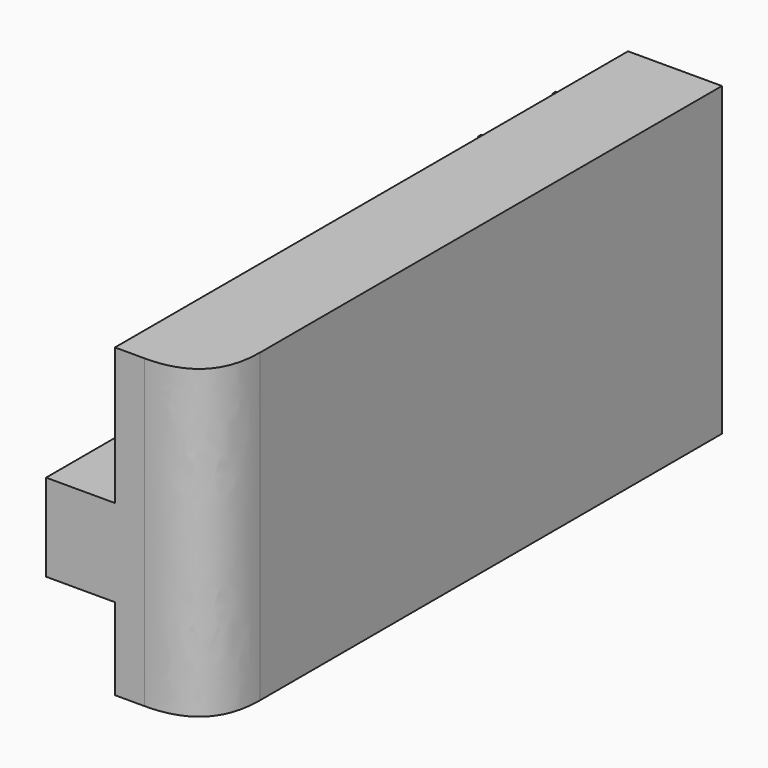
from build123d import *

# Parameters (mm, degrees)
F0_TEXT_SIZE = 35.2777777778
F1_DEPTH     = 2.54
F2_SIZE      = 0.254
F4_DEPTH     = 152.4
F5_T1_DEPTH  = 148.9587342262


# Not quite as in the source:
# - a fillet or chamfer that OpenCascade refuses, or shapes differently, is made with other operations: its cross-section is extruded or revolved along the edge and cut away or added
# - Text() gives the source's letters only with a copy of the font that has no kerning and outlines rounded to 1/6400 em; it was checked with that copy


with BuildPart() as f1:
    # F0 (on Top) → F1 (new body)
    with BuildSketch(Plane.XY):
        with Locations((0, -25.4)):
            Text('M', F0_TEXT_SIZE, font='Tinos', text_align=(TextAlign.LEFT, TextAlign.BOTTOM))
    extrude(amount=F1_DEPTH)

    # F2
    f2_edges = [f1.edges().sort_by_distance(p)[0] for p in [
        (27.373351, -13.841016, 2.54),
        (24.066059, -14.780838, 2.54),
    ]]
    chamfer(f2_edges, length=F2_SIZE)

    # F3 (on Front) → F4 (join)
    with BuildSketch(Plane.XZ):
        Polygon((0, -38.2421910763), (16.3695979863, -38.2421910763), (16.3695979863, -57.7016249299), (38.6810526252, -57.7016249299), (38.6810526252, 15.0571092963), (16.3695979863, 15.0571092963), (16.3695979863, -17.5031870604), (0, -17.5031870604), align=None)
    extrude(amount=F4_DEPTH)

    # F5: fillet of radius 15.24 on 1 edges, made by hand

    # F5_s2 → F5_t1 (cut)
    with BuildSketch(Plane.XY.offset(-95.8016249299)):
        with BuildLine():
            add(Edge.make_bspline(
                [(23.4410526252, -152.4), (38.6810526252, -152.4), (38.6810526252, -137.16)],
                knots=[0, 0, 0, 1, 1, 1], degree=2, weights=[1, 1, 1]))
            Line((38.6810526252, -137.16), (38.6810526252, -152.4))
            Line((38.6810526252, -152.4), (23.4410526252, -152.4))
        make_face()
    extrude(amount=F5_T1_DEPTH, mode=Mode.SUBTRACT)


solid = f1.part
